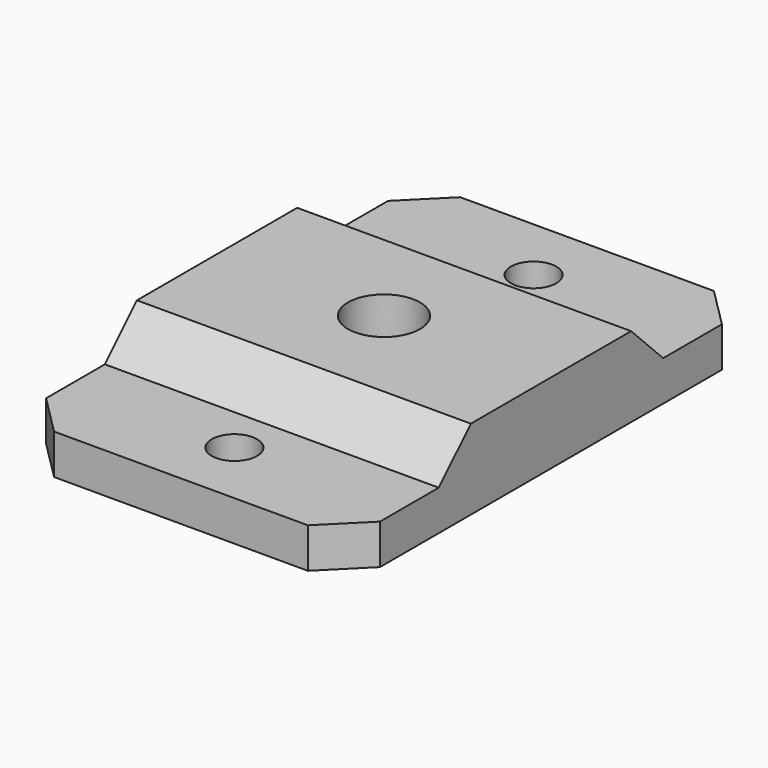
from build123d import *

# Parameters (mm, degrees)
F0_W     = 25
F0_H     = 11.5
F0_R     = 1.7
F1_DEPTH = 3
F0_H_2   = 15
F0_R_2   = 4.6
F0_R_3   = 2.7
F2_DEPTH = 6
F3_DEPTH = 2
F4_SIZE  = 2.99999
F5_START = 2
F5_DEPTH = 0.3


# Not quite as in the source:
# - a fillet or chamfer is up to 0.001 mm smaller than in the source, because OpenCascade refuses the exact size


with BuildPart() as f1:
    # F0 (on Top) → F1 (new body)
    with BuildSketch(Plane.XY):
        with Locations((0, 13.25)):
            Rectangle(F0_W, F0_H)
        with Locations((0, 14)):
            Circle(F0_R, mode=Mode.SUBTRACT)
    extrude(amount=F1_DEPTH)



with BuildPart() as f1b:
    # F0 (on Top) → F1, piece 2 (new body)
    with BuildSketch(Plane.XY):
        with Locations((0, -13.25)):
            Rectangle(F0_W, F0_H)
        with Locations((0, -14)):
            Circle(F0_R, mode=Mode.SUBTRACT)
    extrude(amount=F1_DEPTH)


with BuildPart() as f1_1:
    add(f1.part)

    add(f1b.part)  # F2 merges F1b
    # F0 (on Top) → F2 (join)
    with BuildSketch(Plane.XY):
        Rectangle(F0_W, F0_H_2)
        Circle(F0_R_2, mode=Mode.SUBTRACT)
        Circle(F0_R_2)
        Circle(F0_R_3, mode=Mode.SUBTRACT)
    extrude(amount=F2_DEPTH)

    # F0 (on Top) → F3 (cut)
    with BuildSketch(Plane.XY):
        Circle(F0_R_2)
        Circle(F0_R_3, mode=Mode.SUBTRACT)
    extrude(amount=F3_DEPTH, mode=Mode.SUBTRACT)

    # F4 (size 3 in the source; OpenCascade refuses exactly that, so slightly less here)
    f4_edges = [f1_1.edges().sort_by_distance(p)[0] for p in [
        (0, 7.5, 3),
        (0, -7.5, 3),
        (12.5, -19, 1.5),
        (-12.5, -19, 1.5),
        (12.5, 19, 1.5),
        (-12.5, 19, 1.5),
    ]]
    chamfer(f4_edges, length=F4_SIZE)

    # F0 (on Top) → F5 (join)
    with BuildSketch(Plane.XY.offset(F5_START)):
        Circle(F0_R_3)
    extrude(amount=F5_DEPTH)


solid = f1_1.part
